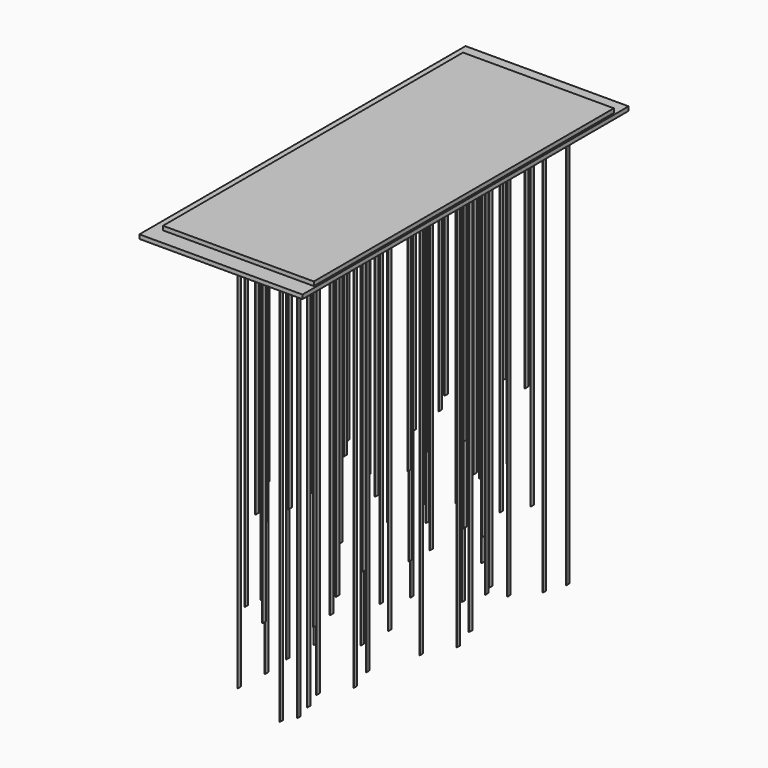
from build123d import *

# Parameters (mm, degrees)
F1_W      = 1
F1_H      = 10
F2_DEPTH  = 1000
F3_W      = 1
F3_H      = 10
F4_DEPTH  = 600
F5_W      = 1
F5_H      = 10
F6_DEPTH  = 800
F7_W      = 400
F7_H      = 1000
F8_DEPTH  = 10
F9_W      = 350
F9_H      = 900
F10_DEPTH = 10
F11_T     = 10


# Not quite as in the source:
# - a feature names something its author has since deleted; it is built from what else it names


with BuildPart() as f2:
    # F1 (on Top) → F2 (new body)
    with BuildSketch(Plane.XY):
        with Locations((135.7242968209, 393.8648324539)):
            Rectangle(F1_W, F1_H)
    extrude(amount=-F2_DEPTH)


with BuildPart() as f2b:
    # F1 (on Top) → F2, piece 2 (new body)
    with BuildSketch(Plane.XY):
        with Locations((119.7553888127, 341.8454080131)):
            Rectangle(F1_W, F1_H)
    extrude(amount=-F2_DEPTH)


with BuildPart() as f2c:
    # F1 (on Top) → F2, piece 3 (new body)
    with BuildSketch(Plane.XY):
        with Locations((-48.3200930826, 364.0674059172)):
            Rectangle(F1_W, F1_H)
    extrude(amount=-F2_DEPTH)


with BuildPart() as f2d:
    # F1 (on Top) → F2, piece 4 (new body)
    with BuildSketch(Plane.XY):
        with Locations((-86.5439306669, 344.0830927421)):
            Rectangle(F1_W, F1_H)
    extrude(amount=-F2_DEPTH)


with BuildPart() as f2e:
    # F1 (on Top) → F2, piece 5 (new body)
    with BuildSketch(Plane.XY):
        with Locations((77.2634587415, 286.285162427)):
            Rectangle(F1_W, F1_H)
    extrude(amount=-F2_DEPTH)


with BuildPart() as f2f:
    # F1 (on Top) → F2, piece 6 (new body)
    with BuildSketch(Plane.XY):
        with Locations((26.6808961682, 293.504002959)):
            Rectangle(F1_W, F1_H)
    extrude(amount=-F2_DEPTH)


with BuildPart() as f2g:
    # F1 (on Top) → F2, piece 7 (new body)
    with BuildSketch(Plane.XY):
        with Locations((39.0396211572, 266.3008492519)):
            Rectangle(F1_W, F1_H)
    extrude(amount=-F2_DEPTH)


with BuildPart() as f2h:
    # F1 (on Top) → F2, piece 8 (new body)
    with BuildSketch(Plane.XY):
        with Locations((23.070713149, 214.2814248111)):
            Rectangle(F1_W, F1_H)
    extrude(amount=-F2_DEPTH)


with BuildPart() as f2i:
    # F1 (on Top) → F2, piece 9 (new body)
    with BuildSketch(Plane.XY):
        with Locations((-65.3622829191, 167.2536437293)):
            Rectangle(F1_W, F1_H)
    extrude(amount=-F2_DEPTH)


with BuildPart() as f2j:
    # F1 (on Top) → F2, piece 10 (new body)
    with BuildSketch(Plane.XY):
        with Locations((-94.5429586641, 109.8894667705)):
            Rectangle(F1_W, F1_H)
    extrude(amount=-F2_DEPTH)


with BuildPart() as f2k:
    # F1 (on Top) → F2, piece 11 (new body)
    with BuildSketch(Plane.XY):
        with Locations((111.4824061446, 125.9487341051)):
            Rectangle(F1_W, F1_H)
    extrude(amount=-F2_DEPTH)


with BuildPart() as f2l:
    # F1 (on Top) → F2, piece 12 (new body)
    with BuildSketch(Plane.XY):
        with Locations((132.8842929728, 61.3657166143)):
            Rectangle(F1_W, F1_H)
    extrude(amount=-F2_DEPTH)


with BuildPart() as f2m:
    # F1 (on Top) → F2, piece 13 (new body)
    with BuildSketch(Plane.XY):
        with Locations((-11.858724989, 32.2031537071)):
            Rectangle(F1_W, F1_H)
    extrude(amount=-F2_DEPTH)


with BuildPart() as f2n:
    # F1 (on Top) → F2, piece 14 (new body)
    with BuildSketch(Plane.XY):
        with Locations((98.1733780354, -8.3048315719)):
            Rectangle(F1_W, F1_H)
    extrude(amount=-F2_DEPTH)


with BuildPart() as f2o:
    # F1 (on Top) → F2, piece 15 (new body)
    with BuildSketch(Plane.XY):
        with Locations((-15.4689080082, -47.0194244408)):
            Rectangle(F1_W, F1_H)
    extrude(amount=-F2_DEPTH)


with BuildPart() as f2p:
    # F1 (on Top) → F2, piece 16 (new body)
    with BuildSketch(Plane.XY):
        with Locations((-87.3357410379, -102.1264917324)):
            Rectangle(F1_W, F1_H)
    extrude(amount=-F2_DEPTH)


with BuildPart() as f2q:
    # F1 (on Top) → F2, piece 17 (new body)
    with BuildSketch(Plane.XY):
        with Locations((-90.9459240571, -181.3490698803)):
            Rectangle(F1_W, F1_H)
    extrude(amount=-F2_DEPTH)


with BuildPart() as f2r:
    # F1 (on Top) → F2, piece 18 (new body)
    with BuildSketch(Plane.XY):
        with Locations((62.2409639113, -127.8294143374)):
            Rectangle(F1_W, F1_H)
    extrude(amount=-F2_DEPTH)


with BuildPart() as f2s:
    # F1 (on Top) → F2, piece 19 (new body)
    with BuildSketch(Plane.XY):
        with Locations((83.6428507395, -192.4124318282)):
            Rectangle(F1_W, F1_H)
    extrude(amount=-F2_DEPTH)


with BuildPart() as f2t:
    # F1 (on Top) → F2, piece 20 (new body)
    with BuildSketch(Plane.XY):
        with Locations((77.8150369572, -358.16020555)):
            Rectangle(F1_W, F1_H)
    extrude(amount=-F2_DEPTH)


with BuildPart() as f2u:
    # F1 (on Top) → F2, piece 21 (new body)
    with BuildSketch(Plane.XY):
        with Locations((64.8584550294, -312.0646444256)):
            Rectangle(F1_W, F1_H)
    extrude(amount=-F2_DEPTH)


with BuildPart() as f2v:
    # F1 (on Top) → F2, piece 22 (new body)
    with BuildSketch(Plane.XY):
        with Locations((61.2482720102, -391.2872225735)):
            Rectangle(F1_W, F1_H)
    extrude(amount=-F2_DEPTH)


with BuildPart() as f2w:
    # F1 (on Top) → F2, piece 23 (new body)
    with BuildSketch(Plane.XY):
        with Locations((-88.5743409231, -333.4139437173)):
            Rectangle(F1_W, F1_H)
    extrude(amount=-F2_DEPTH)


with BuildPart() as f2x:
    # F1 (on Top) → F2, piece 24 (new body)
    with BuildSketch(Plane.XY):
        with Locations((46.5102419533, -260.6712946589)):
            Rectangle(F1_W, F1_H)
    extrude(amount=-F2_DEPTH)


with BuildPart() as f2y:
    # F1 (on Top) → F2, piece 25 (new body)
    with BuildSketch(Plane.XY):
        with Locations((-84.9641579039, -254.1913655694)):
            Rectangle(F1_W, F1_H)
    extrude(amount=-F2_DEPTH)


with BuildPart() as f4:
    # F3 (on Top) → F4 (new body)
    with BuildSketch(Plane.XY):
        with Locations((-57.5457089947, 262.072047929)):
            Rectangle(F3_W, F3_H)
    extrude(amount=-F4_DEPTH)


with BuildPart() as f4b:
    # F3 (on Top) → F4, piece 2 (new body)
    with BuildSketch(Plane.XY):
        with Locations((4.0951761982, -371.1895916959)):
            Rectangle(F3_W, F3_H)
    extrude(amount=-F4_DEPTH)


with BuildPart() as f4c:
    # F3 (on Top) → F4, piece 3 (new body)
    with BuildSketch(Plane.XY):
        with Locations((43.7720023544, 382.2797307048)):
            Rectangle(F3_W, F3_H)
    extrude(amount=-F4_DEPTH)


with BuildPart() as f4d:
    # F3 (on Top) → F4, piece 4 (new body)
    with BuildSketch(Plane.XY):
        with Locations((-0.093400515, -213.6195829835)):
            Rectangle(F3_W, F3_H)
    extrude(amount=-F4_DEPTH)


with BuildPart() as f4e:
    # F3 (on Top) → F4, piece 5 (new body)
    with BuildSketch(Plane.XY):
        with Locations((-10.7687216735, 381.4111265937)):
            Rectangle(F3_W, F3_H)
    extrude(amount=-F4_DEPTH)


with BuildPart() as f4f:
    # F3 (on Top) → F4, piece 6 (new body)
    with BuildSketch(Plane.XY):
        with Locations((83.2732393971, -26.4544791308)):
            Rectangle(F3_W, F3_H)
    extrude(amount=-F4_DEPTH)


with BuildPart() as f4g:
    # F3 (on Top) → F4, piece 7 (new body)
    with BuildSketch(Plane.XY):
        with Locations((100.203202535, -148.1662292381)):
            Rectangle(F3_W, F3_H)
    extrude(amount=-F4_DEPTH)


with BuildPart() as f4h:
    # F3 (on Top) → F4, piece 8 (new body)
    with BuildSketch(Plane.XY):
        with Locations((60.4787370755, 193.0742736558)):
            Rectangle(F3_W, F3_H)
    extrude(amount=-F4_DEPTH)


with BuildPart() as f4i:
    # F3 (on Top) → F4, piece 9 (new body)
    with BuildSketch(Plane.XY):
        with Locations((-32.1988421859, -349.2950016981)):
            Rectangle(F3_W, F3_H)
    extrude(amount=-F4_DEPTH)


with BuildPart() as f4j:
    # F3 (on Top) → F4, piece 10 (new body)
    with BuildSketch(Plane.XY):
        with Locations((3.5167825041, -292.8421611314)):
            Rectangle(F3_W, F3_H)
    extrude(amount=-F4_DEPTH)


with BuildPart() as f4k:
    # F3 (on Top) → F4, piece 11 (new body)
    with BuildSketch(Plane.XY):
        with Locations((89.6594128205, 135.710096697)):
            Rectangle(F3_W, F3_H)
    extrude(amount=-F4_DEPTH)


with BuildPart() as f4l:
    # F3 (on Top) → F4, piece 12 (new body)
    with BuildSketch(Plane.XY):
        with Locations((-86.4205285907, -3.2283496112)):
            Rectangle(F3_W, F3_H)
    extrude(amount=-F4_DEPTH)


with BuildPart() as f4m:
    # F3 (on Top) → F4, piece 13 (new body)
    with BuildSketch(Plane.XY):
        with Locations((-11.8375699967, 317.7902698517)):
            Rectangle(F3_W, F3_H)
    extrude(amount=-F4_DEPTH)


with BuildPart() as f4n:
    # F3 (on Top) → F4, piece 14 (new body)
    with BuildSketch(Plane.XY):
        with Locations((-13.6931519955, 109.9678575993)):
            Rectangle(F3_W, F3_H)
    extrude(amount=-F4_DEPTH)


with BuildPart() as f4o:
    # F3 (on Top) → F4, piece 15 (new body)
    with BuildSketch(Plane.XY):
        with Locations((-97.803413868, -234.3769520521)):
            Rectangle(F3_W, F3_H)
    extrude(amount=-F4_DEPTH)


with BuildPart() as f4p:
    # F3 (on Top) → F4, piece 16 (new body)
    with BuildSketch(Plane.XY):
        with Locations((33.5665158927, -88.9977663755)):
            Rectangle(F3_W, F3_H)
    extrude(amount=-F4_DEPTH)


with BuildPart() as f4q:
    # F3 (on Top) → F4, piece 17 (new body)
    with BuildSketch(Plane.XY):
        with Locations((-25.7167024538, 204.6306282282)):
            Rectangle(F3_W, F3_H)
    extrude(amount=-F4_DEPTH)


with BuildPart() as f4r:
    # F3 (on Top) → F4, piece 18 (new body)
    with BuildSketch(Plane.XY):
        with Locations((-50.9397089481, -54.667789489)):
            Rectangle(F3_W, F3_H)
    extrude(amount=-F4_DEPTH)


with BuildPart() as f4s:
    # F3 (on Top) → F4, piece 19 (new body)
    with BuildSketch(Plane.XY):
        with Locations((62.1031150222, 60.3129118681)):
            Rectangle(F3_W, F3_H)
    extrude(amount=-F4_DEPTH)


with BuildPart() as f4t:
    # F3 (on Top) → F4, piece 20 (new body)
    with BuildSketch(Plane.XY):
        with Locations((-38.0979366601, -165.4220297933)):
            Rectangle(F3_W, F3_H)
    extrude(amount=-F4_DEPTH)


with BuildPart() as f6:
    # F5 (on Top) → F6 (new body)
    with BuildSketch(Plane.XY):
        with Locations((32.2581677167, -185.2039665111)):
            Rectangle(F5_W, F5_H)
    extrude(amount=-F6_DEPTH)


with BuildPart() as f6b:
    # F5 (on Top) → F6, piece 2 (new body)
    with BuildSketch(Plane.XY):
        with Locations((35.8683507359, -105.9813883632)):
            Rectangle(F5_W, F5_H)
    extrude(amount=-F6_DEPTH)


with BuildPart() as f6c:
    # F5 (on Top) → F6, piece 3 (new body)
    with BuildSketch(Plane.XY):
        with Locations((-43.2188483322, -319.5336119506)):
            Rectangle(F5_W, F5_H)
    extrude(amount=-F6_DEPTH)


with BuildPart() as f6d:
    # F5 (on Top) → F6, piece 4 (new body)
    with BuildSketch(Plane.XY):
        with Locations((-44.7579888062, -258.8266830544)):
            Rectangle(F5_W, F5_H)
    extrude(amount=-F6_DEPTH)


with BuildPart() as f6e:
    # F5 (on Top) → F6, piece 5 (new body)
    with BuildSketch(Plane.XY):
        with Locations((106.3578566169, -345.2365345556)):
            Rectangle(F5_W, F5_H)
    extrude(amount=-F6_DEPTH)


with BuildPart() as f6f:
    # F5 (on Top) → F6, piece 6 (new body)
    with BuildSketch(Plane.XY):
        with Locations((99.8044046206, -285.5042282144)):
            Rectangle(F5_W, F5_H)
    extrude(amount=-F6_DEPTH)


with BuildPart() as f6g:
    # F5 (on Top) → F6, piece 7 (new body)
    with BuildSketch(Plane.XY):
        with Locations((87.8154066956, 249.8950787586)):
            Rectangle(F5_W, F5_H)
    extrude(amount=-F6_DEPTH)


with BuildPart() as f6h:
    # F5 (on Top) → F6, piece 8 (new body)
    with BuildSketch(Plane.XY):
        with Locations((118.565201257, 305.9980880817)):
            Rectangle(F5_W, F5_H)
    extrude(amount=-F6_DEPTH)


with BuildPart() as f6i:
    # F5 (on Top) → F6, piece 9 (new body)
    with BuildSketch(Plane.XY):
        with Locations((-55.8590447785, 9.0847884839)):
            Rectangle(F5_W, F5_H)
    extrude(amount=-F6_DEPTH)


with BuildPart() as f6j:
    # F5 (on Top) → F6, piece 10 (new body)
    with BuildSketch(Plane.XY):
        with Locations((-71.8279527867, -42.9346359569)):
            Rectangle(F5_W, F5_H)
    extrude(amount=-F6_DEPTH)


with BuildPart() as f6k:
    # F5 (on Top) → F6, piece 11 (new body)
    with BuildSketch(Plane.XY):
        with Locations((81.1129239952, 43.4604675275)):
            Rectangle(F5_W, F5_H)
    extrude(amount=-F6_DEPTH)


with BuildPart() as f6l:
    # F5 (on Top) → F6, piece 12 (new body)
    with BuildSketch(Plane.XY):
        with Locations((74.4079718931, 155.3194608887)):
            Rectangle(F5_W, F5_H)
    extrude(amount=-F6_DEPTH)


with BuildPart() as f6m:
    # F5 (on Top) → F6, piece 13 (new body)
    with BuildSketch(Plane.XY):
        with Locations((124.9905344663, 148.1006203567)):
            Rectangle(F5_W, F5_H)
    extrude(amount=-F6_DEPTH)


with BuildPart() as f6n:
    # F5 (on Top) → F6, piece 14 (new body)
    with BuildSketch(Plane.XY):
        with Locations((-44.3706890823, 185.8331089442)):
            Rectangle(F5_W, F5_H)
    extrude(amount=-F6_DEPTH)


with BuildPart() as f6o:
    # F5 (on Top) → F6, piece 15 (new body)
    with BuildSketch(Plane.XY):
        with Locations((-0.5930173578, 225.8828638469)):
            Rectangle(F5_W, F5_H)
    extrude(amount=-F6_DEPTH)


with BuildPart() as f6p:
    # F5 (on Top) → F6, piece 16 (new body)
    with BuildSketch(Plane.XY):
        with Locations((19.822923197, -392.6420861507)):
            Rectangle(F5_W, F5_H)
    extrude(amount=-F6_DEPTH)


with BuildPart() as f6q:
    # F5 (on Top) → F6, piece 17 (new body)
    with BuildSketch(Plane.XY):
        with Locations((-49.0183164732, -361.0100362102)):
            Rectangle(F5_W, F5_H)
    extrude(amount=-F6_DEPTH)


with BuildPart() as f6r:
    # F5 (on Top) → F6, piece 18 (new body)
    with BuildSketch(Plane.XY):
        with Locations((-30.9501135274, 336.2211786908)):
            Rectangle(F5_W, F5_H)
    extrude(amount=-F6_DEPTH)


with BuildPart() as f6s:
    # F5 (on Top) → F6, piece 19 (new body)
    with BuildSketch(Plane.XY):
        with Locations((-27.3399305082, 415.4437568387)):
            Rectangle(F5_W, F5_H)
    extrude(amount=-F6_DEPTH)


with BuildPart() as f6t:
    # F5 (on Top) → F6, piece 20 (new body)
    with BuildSketch(Plane.XY):
        with Locations((-50.1127434912, 341.7655324911)):
            Rectangle(F5_W, F5_H)
    extrude(amount=-F6_DEPTH)


with BuildPart() as f6u:
    # F5 (on Top) → F6, piece 21 (new body)
    with BuildSketch(Plane.XY):
        with Locations((78.3619433641, -17.1369866002)):
            Rectangle(F5_W, F5_H)
    extrude(amount=-F6_DEPTH)


with BuildPart() as f6v:
    # F5 (on Top) → F6, piece 22 (new body)
    with BuildSketch(Plane.XY):
        with Locations((-104.4618785381, -80.6013923138)):
            Rectangle(F5_W, F5_H)
    extrude(amount=-F6_DEPTH)


with BuildPart() as f6w:
    # F5 (on Top) → F6, piece 23 (new body)
    with BuildSketch(Plane.XY):
        with Locations((-54.5722469687, 83.3180993795)):
            Rectangle(F5_W, F5_H)
    extrude(amount=-F6_DEPTH)


with BuildPart() as f6x:
    # F5 (on Top) → F6, piece 24 (new body)
    with BuildSketch(Plane.XY):
        with Locations((4.4953976758, 126.7966926098)):
            Rectangle(F5_W, F5_H)
    extrude(amount=-F6_DEPTH)


with BuildPart() as f6y:
    # F5 (on Top) → F6, piece 25 (new body)
    with BuildSketch(Plane.XY):
        with Locations((-10.1330308244, -141.1252841353)):
            Rectangle(F5_W, F5_H)
    extrude(amount=-F6_DEPTH)


with BuildPart() as f6z:
    # F5 (on Top) → F6, piece 26 (new body)
    with BuildSketch(Plane.XY):
        with Locations((61.2295679748, -219.0656512976)):
            Rectangle(F5_W, F5_H)
    extrude(amount=-F6_DEPTH)


with BuildPart() as f8:
    # F7 (on Top) → F8 (new body)
    with BuildSketch(Plane.XY):
        Rectangle(F7_W, F7_H)
    extrude(amount=F8_DEPTH)


with BuildPart() as f10:
    # F9 (on Top) → F10 (new body)
    with BuildSketch(Plane.XY):
        with Locations((10.0405421108, 1.0375299025)):
            Rectangle(F9_W, F9_H)
    extrude(amount=F10_DEPTH)

    # F11
    f11_openings = [f10.faces().sort_by_distance(p)[0] for p in [
        (10.040542, 1.03753, 0),
    ]]
    offset(amount=F11_T, openings=f11_openings, kind=Kind.INTERSECTION)


solid = Compound([f2.part, f2b.part, f2c.part, f2d.part, f2e.part, f2f.part, f2g.part, f2h.part, f2i.part, f2j.part, f2k.part, f2l.part, f2m.part, f2n.part, f2o.part, f2p.part, f2q.part, f2r.part, f2s.part, f2t.part, f2u.part, f2v.part, f2w.part, f2x.part, f2y.part, f4.part, f4b.part, f4c.part, f4d.part, f4e.part, f4f.part, f4g.part, f4h.part, f4i.part, f4j.part, f4k.part, f4l.part, f4m.part, f4n.part, f4o.part, f4p.part, f4q.part, f4r.part, f4s.part, f4t.part, f6.part, f6b.part, f6c.part, f6d.part, f6e.part, f6f.part, f6g.part, f6h.part, f6i.part, f6j.part, f6k.part, f6l.part, f6m.part, f6n.part, f6o.part, f6p.part, f6q.part, f6r.part, f6s.part, f6t.part, f6u.part, f6v.part, f6w.part, f6x.part, f6y.part, f6z.part, f8.part, f10.part])
